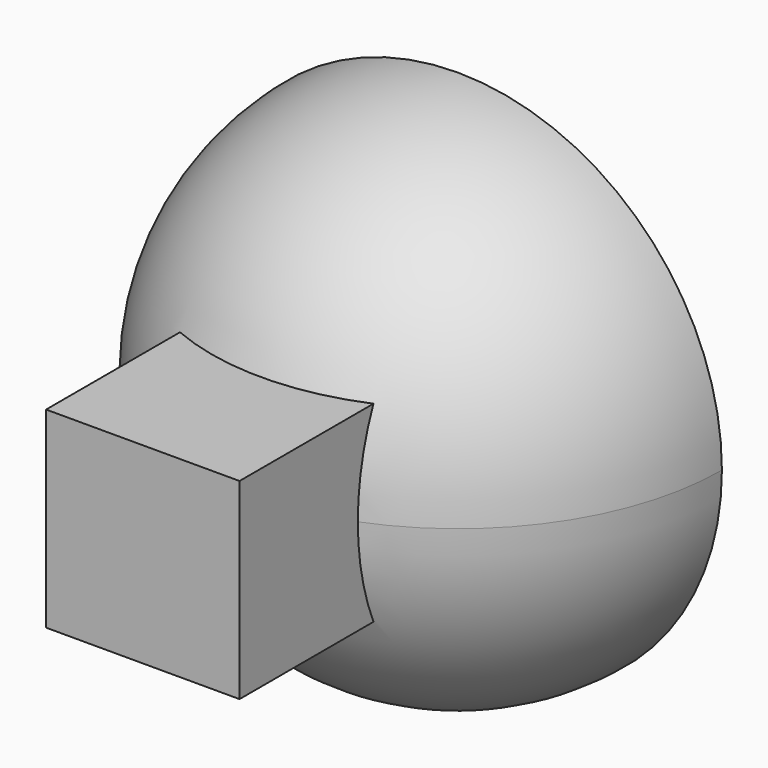
from build123d import *

# Parameters (mm, degrees)
F1_ANGLE = 180
F2_T     = -2.5
F4_W     = 39.3107756972
F4_H     = 39.0258319676


with BuildPart() as f1:
    # F0 (on Front) → F1 (revolve)
    with BuildSketch(Plane.XZ):
        with BuildLine():
            ThreePointArc((0, -53.6816862102), (37.9586843448, -37.9586843448), (53.6816862102, 0))
            ThreePointArc((53.6816862102, 0), (37.9586843448, 37.9586843448), (0, 53.6816862102))
            Line((0, 53.6816862102), (0, -53.6816862102))
        make_face()
    revolve(axis=Axis((0, 0, 0), (0, 0, -1)), revolution_arc=F1_ANGLE)

    # F2
    f2_openings = [f1.faces().sort_by_distance(p)[0] for p in [
        (0, 0, 0),
    ]]
    offset(amount=F2_T, openings=f2_openings)

    # F4 (on offset) → F5 (join, up to the next surface of F1)
    with BuildSketch(Plane.XZ.offset(80)):
        Rectangle(F4_W, F4_H)
    extrude(until=Until.NEXT, dir=(0, 1, 0))


solid = f1.part
